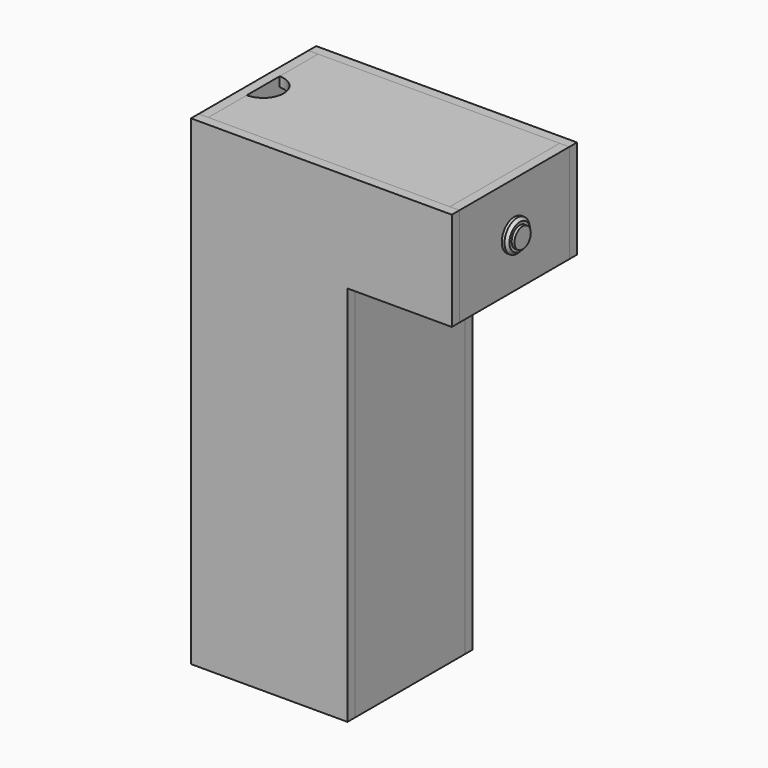
from build123d import *

# Parameters (mm, degrees)
F0_W           = 100
F0_H           = 100
F1_DEPTH       = 7
F3_DEPTH       = 7
F4_START       = -100
F4_DEPTH       = 7
F5_W           = 100
F5_H           = 278
F6_DEPTH       = 7
F7_W           = 100
F7_H           = 343
F8_DEPTH       = 7
F9_W           = 100
F9_H           = 72
F9_R           = 10
F10_DEPTH      = 7
F12_DEPTH      = 7
F13_W          = 76
F13_H          = 100
F13_R          = 5
F14_DEPTH      = 7
F17_R          = 7.4
F18_DEPTH      = 2
F18_DEPTH_BACK = 10
F19_R          = 4.75
F19_R_2        = 3.75
F20_DEPTH      = 25
F20_DEPTH_BACK = 7
F22_DEPTH      = 7


with BuildPart() as f1:
    # F0 (on Top) → F1 (new body)
    with BuildSketch(Plane.XY):
        Rectangle(F0_W, F0_H)
    extrude(amount=F1_DEPTH)


with BuildPart() as f3:
    # F2 (on face) → F3 (new body)
    with BuildSketch(Plane(origin=(0, 50, 0), x_dir=(-1, 0, 0), z_dir=(0, 1, 0))):
        Polygon((-57, 278), (-57, 0), (57, 0), (57, 350), (-133, 350), (-133, 278), align=None)
    extrude(amount=F3_DEPTH)


with BuildPart() as f4:
    # F2 (on face) → F4 (new body)
    with BuildSketch(Plane(origin=(0, 50, 0), x_dir=(-1, 0, 0), z_dir=(0, 1, 0)).offset(F4_START)):
        Polygon((-57, 278), (-57, 0), (57, 0), (57, 350), (-133, 350), (-133, 278), align=None)
    extrude(amount=-F4_DEPTH)


with BuildPart() as f6:
    # F5 (on face) → F6 (new body)
    with BuildSketch(Plane.YZ.offset(50)):
        with Locations((0, 139)):
            Rectangle(F5_W, F5_H)
    extrude(amount=F6_DEPTH)


with BuildPart() as f8:
    # F7 (on face) → F8 (new body)
    with BuildSketch(Plane(origin=(-50, 0, 0), x_dir=(0, -1, 0), z_dir=(-1, 0, 0))):
        with Locations((0, 178.5)):
            Rectangle(F7_W, F7_H)
    extrude(amount=F8_DEPTH)


with BuildPart() as f10:
    # F9 (on face) → F10 (new body)
    with BuildSketch(Plane.YZ.offset(133)):
        with Locations((0, 314)):
            Rectangle(F9_W, F9_H)
        with Locations((0, 314)):
            Circle(F9_R, mode=Mode.SUBTRACT)
    extrude(amount=-F10_DEPTH)


with BuildPart() as f12:
    # F11 (on face) → F12 (new body)
    with BuildSketch(Plane.XY.offset(350)):
        with BuildLine():
            Line((-50, -15), (-50, -50))
            Line((-50, -50), (126, -50))
            Line((126, -50), (126, 50))
            Line((126, 50), (-50, 50))
            Line((-50, 50), (-50, 15))
            ThreePointArc((-50, 15), (-39.3933982822, 10.6066017178), (-35, 0))
            ThreePointArc((-35, 0), (-39.3933982822, -10.6066017178), (-50, -15))
        make_face()
    extrude(amount=-F12_DEPTH)


with BuildPart() as f14:
    # F13 (on face) → F14 (new body)
    with BuildSketch(Plane(origin=(0, 0, 278), x_dir=(1, 0, 0), z_dir=(0, 0, -1))):
        with Locations((88, 0)):
            Rectangle(F13_W, F13_H)
        with Locations((91.5, 0)):
            Circle(F13_R, mode=Mode.SUBTRACT)
    extrude(amount=-F14_DEPTH)


with BuildPart() as f16:
    # F15 (on Front) → F16 (revolve)
    with BuildSketch(Plane.XZ):
        Polygon((133, 325.5), (133, 323.5), (107, 323.5), (107, 314), (111, 314), (111, 321.5), (137, 321.5), (137, 323.5), (135, 325.5), align=None)
    revolve(axis=Axis((109, 0, 314), (-1, 0, 0)))


with BuildPart() as f18:
    # F17 (on face) → F18 (new body, two sides)
    with BuildSketch(Plane.YZ.offset(137)) as f18_sk:
        with Locations((0, 314)):
            Circle(F17_R)
    extrude(amount=F18_DEPTH)
    extrude(f18_sk.sketch, amount=-F18_DEPTH_BACK)


with BuildPart() as f20:
    # F19 (on face) → F20 (new body, two sides)
    with BuildSketch(Plane(origin=(0, 0, 278), x_dir=(1, 0, 0), z_dir=(0, 0, -1))) as f20_sk:
        with Locations((91.5, 0)):
            Circle(F19_R)
        with Locations((91.5, 0)):
            Circle(F19_R_2, mode=Mode.SUBTRACT)
    extrude(amount=F20_DEPTH)
    extrude(f20_sk.sketch, amount=-F20_DEPTH_BACK)


with BuildPart() as f22:
    # F21 (on face) → F22 (new body)
    with BuildSketch(Plane(origin=(0, 0, 343), x_dir=(1, 0, 0), z_dir=(0, 0, -1))):
        with BuildLine():
            ThreePointArc((50, 0), (35.3553390593, -35.3553390593), (0, -50))
            Line((0, -50), (126, -50))
            Line((126, -50), (126, -35))
            Line((126, -35), (76, -35))
            Line((76, -35), (76, 35))
            Line((76, 35), (126, 35))
            Line((126, 35), (126, 50))
            Line((126, 50), (3.1482449267, 50))
            Line((3.1482449267, 50), (6.44e-08, 50))
            ThreePointArc((6.44e-08, 50), (35.3553390821, 35.3553390366), (50, 0))
        make_face()
    extrude(amount=F22_DEPTH)


solid = Compound([f1.part, f3.part, f4.part, f6.part, f8.part, f10.part, f12.part, f14.part, f16.part, f18.part, f20.part, f22.part])
